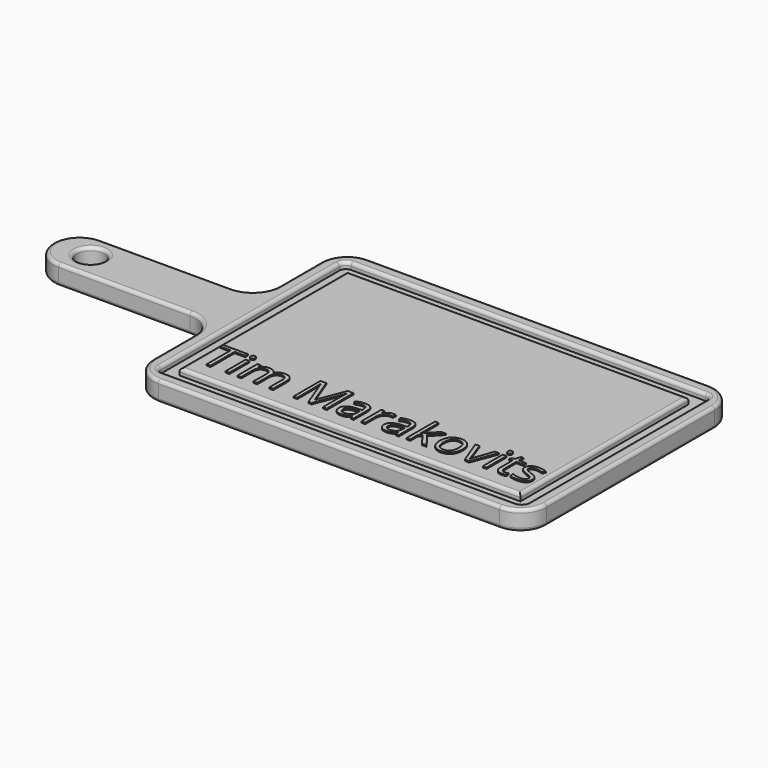
from build123d import *

# Parameters (mm, degrees)
F0_W         = 177.8
F0_H         = 50.8
F1_DEPTH     = 19.05
F2_R         = 13.335
F3_DEPTH     = 228.6
F5_DEPTH     = 6.35
F6_R         = 6.35
F7_R         = 25.39999
F8_R         = 3.175
F9_TEXT_SIZE = 45.2857891977
F10_DEPTH    = 1.27


# Not quite as in the source:
# - a fillet or chamfer is up to 0.001 mm smaller than in the source, because OpenCascade refuses the exact size
# - Text() gives the source's letters only with a copy of the font that has no kerning and outlines rounded to 1/6400 em; it was checked with that copy


with BuildPart() as f1:
    # F0 (on Top) → F1 (new body)
    with BuildSketch(Plane.XY):
        Polygon((0, 101.6), (0, 0), (381, 0), (381, 254), (0, 254), (0, 152.4), align=None)
        with Locations((-88.9, 127)):
            Rectangle(F0_W, F0_H)
    extrude(amount=F1_DEPTH)

    # F2 (on face) → F3 (cut)
    with BuildSketch(Plane.XY.offset(19.05)):
        with Locations((-142.2218233347, 127.635)):
            Circle(F2_R)
    extrude(amount=-F3_DEPTH, mode=Mode.SUBTRACT)

    # F4 (on face) → F5 (cut)
    with BuildSketch(Plane.XY.offset(19.05)):
        Polygon((12.7, 101.6), (12.7, 12.7), (368.3, 12.7), (368.3, 241.3), (12.7, 241.3), (12.7, 152.4), align=None)
        Polygon((25.4, 101.6), (25.4, 152.4), (25.4, 228.6), (355.6, 228.6), (355.6, 25.4), (25.4, 25.4), align=None, mode=Mode.SUBTRACT)
    extrude(amount=-F5_DEPTH, mode=Mode.SUBTRACT)

    # F6
    f6_edges = [f1.edges().sort_by_distance(p)[0] for p in [
        (12.7, 241.3, 15.875),
        (368.3, 241.3, 15.875),
        (368.3, 12.7, 15.875),
        (12.7, 12.7, 15.875),
    ]]
    fillet(f6_edges, radius=F6_R)

    # F7 (radius 25.4 in the source; OpenCascade refuses exactly that, so slightly less here)
    f7_edges = [f1.edges().sort_by_distance(p)[0] for p in [
        (-177.8, 101.6, 9.525),
        (-177.8, 152.4, 9.525),
        (0, 152.4, 9.525),
        (0, 254, 9.525),
        (0, 0, 9.525),
        (0, 101.6, 9.525),
        (381, 0, 9.525),
        (381, 254, 9.525),
    ]]
    fillet(f7_edges, radius=F7_R)

    # F8
    f8_edges = [f1.edges().sort_by_distance(p)[0] for p in [
        (190.5, 228.6, 19.05),
        (355.6, 127, 19.05),
        (190.5, 25.4, 19.05),
        (25.4, 127, 19.05),
        (0, 50.8, 19.05),
        (-7.439485, 94.160515, 19.05),
        (7.439485, 7.439485, 19.05),
        (-88.9, 101.6, 19.05),
        (190.5, 0, 19.05),
        (-170.360515, 109.039485, 19.05),
        (373.560515, 7.439485, 19.05),
        (-177.8, 127, 19.05),
        (381, 127, 19.05),
        (-170.360515, 144.960515, 19.05),
        (373.560515, 246.560515, 19.05),
        (-88.9, 152.4, 19.05),
        (190.5, 254, 19.05),
        (-7.439485, 159.839485, 19.05),
        (7.439485, 246.560515, 19.05),
        (0, 203.2, 19.05),
        (190.5, 12.7, 19.05),
        (14.559872, 14.559872, 19.05),
        (366.440128, 14.559872, 19.05),
        (12.7, 127, 19.05),
        (368.3, 127, 19.05),
        (14.559872, 239.440128, 19.05),
        (366.440128, 239.440128, 19.05),
        (190.5, 241.3, 19.05),
        (-155.556823, 127.635, 19.05),
        (0, 50.8, 0),
        (-7.439485, 94.160515, 0),
        (7.439485, 7.439485, 0),
        (-88.9, 101.6, 0),
        (190.5, 0, 0),
        (-170.360515, 109.039485, 0),
        (373.560515, 7.439485, 0),
        (-177.8, 127, 0),
        (381, 127, 0),
        (-170.360515, 144.960515, 0),
        (373.560515, 246.560515, 0),
        (-88.9, 152.4, 0),
        (190.5, 254, 0),
        (-7.439485, 159.839485, 0),
        (7.439485, 246.560515, 0),
        (0, 203.2, 0),
        (-155.556823, 127.635, 0),
    ]]
    fillet(f8_edges, radius=F8_R)

    # F9 (on face) → F10 (join)
    with BuildSketch(Plane.XY.offset(19.05)):
        with Locations((28.575, 41.275)):
            Text('Tim Marakovits', F9_TEXT_SIZE, font='Open Sans', text_align=(TextAlign.LEFT, TextAlign.BOTTOM))
    extrude(amount=F10_DEPTH)


solid = f1.part
